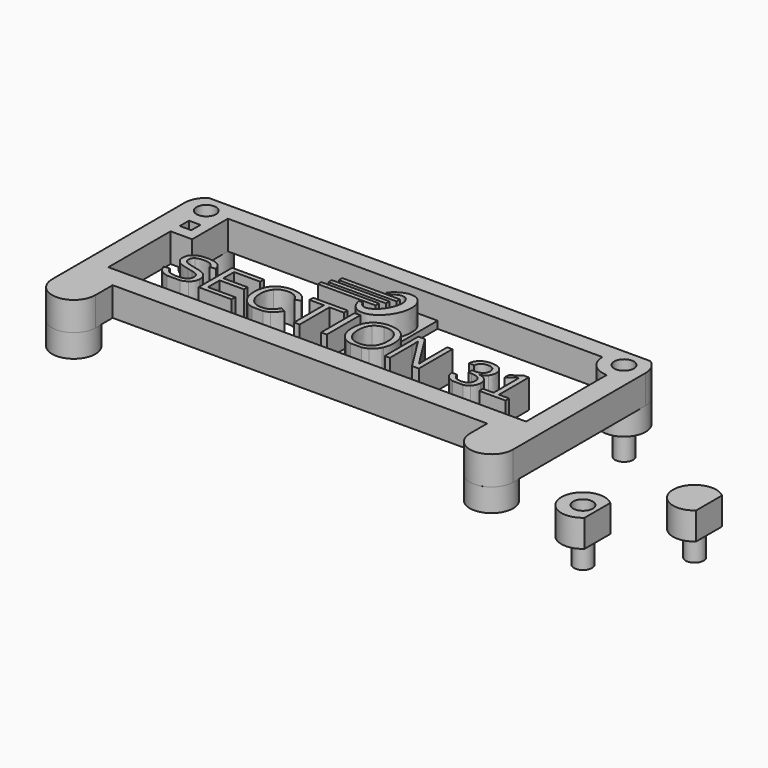
from build123d import *

# Parameters (mm, degrees)
F0_R      = 1.25
F1_DEPTH  = 3.8
F3_DEPTH  = 3.2
F0_R_2    = 3
F0_R_3    = 1.35
F4_W      = 0.7852271802
F4_H      = 1.481747925
F4_W_2    = 0.789192974
F4_W_3    = 0.7019455096
F4_H_2    = 4.3387154998
F4_W_4    = 0.7194174142
F4_H_3    = 0.6437805332
F4_W_5    = 2.3355792606
F4_H_4    = 0.6
F4_W_6    = 2.9250326228
F4_W_7    = 3.514485985
F5_DEPTH  = 1
F4_W_8    = 52
F4_H_5    = 3
F6_DEPTH  = 4
F4_W_9    = 5.6644207394
F4_W_10   = 5.0749673772
F4_W_11   = 4.485514015
F7_DEPTH  = 4
F8_R      = 1.35
F9_DEPTH  = 3
F10_DEPTH = 3.5
F2_R      = 1
F11_R     = 1.35
F11_R_2   = 1
F12_DEPTH = 2.5


with BuildPart() as f1:
    # F0 (on Top) → F1 (new body)
    with BuildSketch(Plane.XY):
        with BuildLine():
            Line((2, -2.2360679775), (2, 2.2360679775))
            ThreePointArc((2, 2.2360679775), (-3, 0), (2, -2.2360679775))
        make_face()
        Circle(F0_R, mode=Mode.SUBTRACT)
        Circle(F0_R)
    extrude(amount=F1_DEPTH)

    # F0 (on Top) → F10 (join)
    with BuildSketch(Plane.XY):
        Circle(F0_R)
    extrude(amount=-F10_DEPTH)

    # F2 (on face) + F11 (on face) → F12 (cut)
    with BuildSketch(Plane.XY.offset(3.8)):
        Circle(F2_R)
    with BuildSketch(Plane.XY.offset(3.8)):
        Circle(F11_R)
        Circle(F11_R_2, mode=Mode.SUBTRACT)
    extrude(amount=-F12_DEPTH, mode=Mode.SUBTRACT)


with BuildPart() as f1b:
    # F0 (on Top) → F1, piece 2 (new body)
    with BuildSketch(Plane.XY):
        with BuildLine():
            Line((10.3669340588, 6.6795249388), (10.3669340588, 11.1516608938))
            ThreePointArc((10.3669340588, 11.1516608938), (5.3669340588, 8.9155929163), (10.3669340588, 6.6795249388))
        make_face()
        with Locations((8.3669340588, 8.9155929163)):
            Circle(F0_R, mode=Mode.SUBTRACT)
        with Locations((8.3669340588, 8.9155929163)):
            Circle(F0_R)
    extrude(amount=F1_DEPTH)


with BuildPart() as f3:
    # F0 (on Top) → F3 (new body)
    with BuildSketch(Plane.XY):
        with BuildLine():
            Line((-11.3286585063, 25.8566533644), (-14.6452832967, 25.8566533644))
            ThreePointArc((-14.6452832967, 25.8566533644), (-12.9869709015, 20.3566533644), (-11.3286585063, 25.8566533644))
        make_face()
        with Locations((-12.9869709015, 23.3566533644)):
            Circle(F0_R, mode=Mode.SUBTRACT)
        with Locations((-12.9869709015, 23.3566533644)):
            Circle(F0_R)
    extrude(amount=F3_DEPTH)


with BuildPart() as f3b:
    # F0 (on Top) → F3, piece 2 (new body)
    with BuildSketch(Plane.XY):
        with BuildLine():
            Line((-69.3286585063, 25.8566533644), (-72.6452832967, 25.8566533644))
            ThreePointArc((-72.6452832967, 25.8566533644), (-70.9869709015, 20.3566533644), (-69.3286585063, 25.8566533644))
        make_face()
        with Locations((-70.9869709015, 23.3566533644)):
            Circle(F0_R, mode=Mode.SUBTRACT)
        with Locations((-70.9869709015, 23.3566533644)):
            Circle(F0_R)
    extrude(amount=F3_DEPTH)


with BuildPart() as f3c:
    # F0 (on Top) → F3, piece 3 (new body)
    with BuildSketch(Plane.XY):
        with Locations((-70.9869709015, 0.3566533644)):
            Circle(F0_R_2)
        with Locations((-70.9869709015, 0.3566533644)):
            Circle(F0_R_3, mode=Mode.SUBTRACT)
    extrude(amount=F3_DEPTH)


with BuildPart() as f3d:
    # F0 (on Top) → F3, piece 4 (new body)
    with BuildSketch(Plane.XY):
        with Locations((-12.9869709015, 0.3566533644)):
            Circle(F0_R_2)
        with Locations((-12.9869709015, 0.3566533644)):
            Circle(F0_R_3, mode=Mode.SUBTRACT)
    extrude(amount=F3_DEPTH)


with BuildPart() as f5:
    # F4 (on face) → F5 (new body)
    with BuildSketch(Plane.XY.offset(3.2)):
        with BuildLine():
            Line((-65.9445128975, 10.2926716208), (-70.9869709015, 10.2926716208))
            Line((-70.9869709015, 10.2926716208), (-70.9869709015, 8.8109236958))
            Line((-70.9869709015, 8.8109236958), (-64.8152467128, 8.8109236958))
            add(Edge.make_bspline(
                [(-64.8152467128, 8.8109236958), (-66.1138597254, 9.0786315838), (-66.3719762536, 10.2068831272)],
                knots=[0.2372767753, 0.2372767753, 0.2372767753, 1, 1, 1], degree=2))
            Line((-66.3719762536, 10.2068831272), (-65.9445128975, 10.2926716208))
        make_face()
        with BuildLine():
            Line((-65.58930585, 10.2926716208), (-65.9445128975, 10.2926716208))
            Line((-65.9445128975, 10.2926716208), (-66.3719762536, 10.2068831272))
            add(Edge.make_bspline(
                [(-64.8152467128, 8.8109236958), (-66.1138597254, 9.0786315838), (-66.3719762536, 10.2068831272)],
                knots=[0.2372767753, 0.2372767753, 0.2372767753, 1, 1, 1], degree=2))
            Line((-64.8152467128, 8.8109236958), (-63.0099098319, 8.8109236958))
            add(Edge.make_bspline(
                [(-62.1318816738, 9.1698280383), (-62.4884162435, 8.919543015), (-63.0099098319, 8.8109236958)],
                knots=[0, 0, 0, 0.5660175036, 0.5660175036, 0.5660175036], degree=2))
            add(Edge.make_bspline(
                [(-61.5059502002, 10.2926716208), (-61.5519807819, 9.5769148133), (-62.1318816738, 9.1698280383)],
                knots=[0.0793766355, 0.0793766355, 0.0793766355, 1, 1, 1], degree=2))
            Line((-61.5059502002, 10.2926716208), (-62.2861622514, 10.2926716208))
            add(Edge.make_bspline(
                [(-62.6983292272, 9.6060653606), (-62.3180540452, 9.8464622511), (-62.2861622514, 10.2926716208)],
                knots=[0, 0, 0, 0.9161349587, 0.9161349587, 0.9161349587], degree=2))
            add(Edge.make_bspline(
                [(-63.8774919287, 9.3436620015), (-63.113415649, 9.3436620015), (-62.6983292272, 9.6060653606)],
                knots=[0, 0, 0, 1, 1, 1], degree=2))
            add(Edge.make_bspline(
                [(-65.04607918, 9.5895412196), (-64.6164515141, 9.3436620015), (-63.8774919287, 9.3436620015)],
                knots=[0, 0, 0, 1, 1, 1], degree=2))
            add(Edge.make_bspline(
                [(-65.58930585, 10.2926716208), (-65.4475651637, 9.8193147364), (-65.04607918, 9.5895412196)],
                knots=[0.0655024909, 0.0655024909, 0.0655024909, 1, 1, 1], degree=2))
        make_face()
        with BuildLine():
            Line((-62.2861622514, 10.2926716208), (-65.58930585, 10.2926716208))
            add(Edge.make_bspline(
                [(-65.58930585, 10.2926716208), (-65.4475651637, 9.8193147364), (-65.04607918, 9.5895412196)],
                knots=[0.0655024909, 0.0655024909, 0.0655024909, 1, 1, 1], degree=2))
            add(Edge.make_bspline(
                [(-65.04607918, 9.5895412196), (-64.6164515141, 9.3436620015), (-63.8774919287, 9.3436620015)],
                knots=[0, 0, 0, 1, 1, 1], degree=2))
            add(Edge.make_bspline(
                [(-63.8774919287, 9.3436620015), (-63.113415649, 9.3436620015), (-62.6983292272, 9.6060653606)],
                knots=[0, 0, 0, 1, 1, 1], degree=2))
            add(Edge.make_bspline(
                [(-62.6983292272, 9.6060653606), (-62.3180540452, 9.8464622511), (-62.2861622514, 10.2926716208)],
                knots=[0, 0, 0, 0.9161349587, 0.9161349587, 0.9161349587], degree=2))
        make_face()
        with BuildLine():
            add(Edge.make_bspline(
                [(-62.1318816738, 9.1698280383), (-62.4884162435, 8.919543015), (-63.0099098319, 8.8109236958)],
                knots=[0, 0, 0, 0.5660175036, 0.5660175036, 0.5660175036], degree=2))
            Line((-63.0099098319, 8.8109236958), (-60.4193197009, 8.8109236958))
            Line((-60.4193197009, 8.8109236958), (-60.4193197009, 10.2926716208))
            Line((-60.4193197009, 10.2926716208), (-61.5059502002, 10.2926716208))
            add(Edge.make_bspline(
                [(-61.5059502002, 10.2926716208), (-61.5519807819, 9.5769148133), (-62.1318816738, 9.1698280383)],
                knots=[0.0793766355, 0.0793766355, 0.0793766355, 1, 1, 1], degree=2))
        make_face()
        Polygon((-60.4193197009, 10.2926716208), (-60.4193197009, 8.8109236958), (-55.8335400914, 8.8109236958), (-55.8335400914, 9.4560261603), (-59.6301267269, 9.4560261603), (-59.6301267269, 10.2926716208), align=None)
        with BuildLine():
            Line((-55.8335400914, 9.4560261603), (-55.8335400914, 8.8109236958))
            Line((-55.8335400914, 8.8109236958), (-52.9878142088, 8.8109236958))
            add(Edge.make_bspline(
                [(-52.9878142088, 8.8109236958), (-53.3889917697, 8.9022720993), (-53.7250597001, 9.0938169897)],
                knots=[0.4769033687, 0.4769033687, 0.4769033687, 1, 1, 1], degree=2))
            add(Edge.make_bspline(
                [(-53.7250597001, 9.0938169897), (-54.3675183021, 9.4599919542), (-54.7039498128, 10.139464632)],
                knots=[0, 0, 0, 1, 1, 1], degree=2))
            add(Edge.make_bspline(
                [(-54.7039498128, 10.139464632), (-54.7411237954, 10.2145429308), (-54.7741902407, 10.2926716208)],
                knots=[0, 0, 0, 0.110494949, 0.110494949, 0.110494949], degree=2))
            Line((-54.7741902407, 10.2926716208), (-59.6301267269, 10.2926716208))
            Line((-59.6301267269, 10.2926716208), (-59.6301267269, 9.4560261603))
            Line((-59.6301267269, 9.4560261603), (-55.8335400914, 9.4560261603))
        make_face()
        with BuildLine():
            add(Edge.make_bspline(
                [(-52.9878142088, 8.8109236958), (-53.3889917697, 8.9022720993), (-53.7250597001, 9.0938169897)],
                knots=[0.4769033687, 0.4769033687, 0.4769033687, 1, 1, 1], degree=2))
            Line((-52.9878142088, 8.8109236958), (-51.4550116902, 8.8109236958))
            add(Edge.make_bspline(
                [(-50.6925493444, 9.1202556153), (-51.0433918047, 8.9084665691), (-51.4550116902, 8.8109236958)],
                knots=[0, 0, 0, 0.5394338135, 0.5394338135, 0.5394338135], degree=2))
            add(Edge.make_bspline(
                [(-49.6825938466, 10.2650481035), (-50.0421591547, 9.5128692054), (-50.6925493444, 9.1202556153)],
                knots=[0, 0, 0, 1, 1, 1], degree=2))
            Line((-49.6825938466, 10.2650481035), (-49.7377276701, 10.2926716208))
            Line((-49.7377276701, 10.2926716208), (-50.4971638043, 10.2926716208))
            add(Edge.make_bspline(
                [(-52.16518079, 9.3767102835), (-51.101681984, 9.3767102835), (-50.4971638043, 10.2926716208)],
                knots=[0, 0, 0, 0.8697338936, 0.8697338936, 0.8697338936], degree=2))
            add(Edge.make_bspline(
                [(-53.679453071, 10.0277614388), (-53.119615174, 9.3767102835), (-52.16518079, 9.3767102835)],
                knots=[0, 0, 0, 1, 1, 1], degree=2))
            add(Edge.make_bspline(
                [(-53.8734730775, 10.2926716208), (-53.7867440439, 10.1525331133), (-53.679453071, 10.0277614388)],
                knots=[0.8083535011, 0.8083535011, 0.8083535011, 1, 1, 1], degree=2))
            Line((-53.8734730775, 10.2926716208), (-54.7741902407, 10.2926716208))
            add(Edge.make_bspline(
                [(-54.7039498128, 10.139464632), (-54.7411237954, 10.2145429308), (-54.7741902407, 10.2926716208)],
                knots=[0, 0, 0, 0.110494949, 0.110494949, 0.110494949], degree=2))
            add(Edge.make_bspline(
                [(-53.7250597001, 9.0938169897), (-54.3675183021, 9.4599919542), (-54.7039498128, 10.139464632)],
                knots=[0, 0, 0, 1, 1, 1], degree=2))
        make_face()
        with BuildLine():
            add(Edge.make_bspline(
                [(-52.16518079, 9.3767102835), (-51.101681984, 9.3767102835), (-50.4971638043, 10.2926716208)],
                knots=[0, 0, 0, 0.8697338936, 0.8697338936, 0.8697338936], degree=2))
            Line((-50.4971638043, 10.2926716208), (-53.8734730775, 10.2926716208))
            add(Edge.make_bspline(
                [(-53.8734730775, 10.2926716208), (-53.7867440439, 10.1525331133), (-53.679453071, 10.0277614388)],
                knots=[0.8083535011, 0.8083535011, 0.8083535011, 1, 1, 1], degree=2))
            add(Edge.make_bspline(
                [(-53.679453071, 10.0277614388), (-53.119615174, 9.3767102835), (-52.16518079, 9.3767102835)],
                knots=[0, 0, 0, 1, 1, 1], degree=2))
        make_face()
        with BuildLine():
            Line((-47.1709244151, 8.8109236958), (-47.1709244151, 10.2926716208))
            Line((-47.1709244151, 10.2926716208), (-49.7377276701, 10.2926716208))
            Line((-49.7377276701, 10.2926716208), (-49.6825938466, 10.2650481035))
            add(Edge.make_bspline(
                [(-49.6825938466, 10.2650481035), (-50.0421591547, 9.5128692054), (-50.6925493444, 9.1202556153)],
                knots=[0, 0, 0, 1, 1, 1], degree=2))
            add(Edge.make_bspline(
                [(-50.6925493444, 9.1202556153), (-51.0433918047, 8.9084665691), (-51.4550116902, 8.8109236958)],
                knots=[0, 0, 0, 0.5394338135, 0.5394338135, 0.5394338135], degree=2))
            Line((-51.4550116902, 8.8109236958), (-47.1709244151, 8.8109236958))
        make_face()
        with Locations((-46.778310825, 9.5517976583)):
            Rectangle(F4_W, F4_H)
        Polygon((-43.4113518554, 8.8109236958), (-43.4113518554, 10.2926716208), (-45.1050326228, 10.2926716208), (-46.3856972349, 10.2926716208), (-46.3856972349, 8.8109236958), align=None)
        with Locations((-43.0167553684, 9.5517976583)):
            Rectangle(F4_W_2, F4_H)
        with BuildLine():
            add(Edge.make_bspline(
                [(-41.0986330815, 10.1434304258), (-41.1352188102, 10.2167428687), (-41.1679026296, 10.2926716208)],
                knots=[0, 0, 0, 0.1066511318, 0.1066511318, 0.1066511318], degree=2))
            Line((-41.1679026296, 10.2926716208), (-42.6221588814, 10.2926716208))
            Line((-42.6221588814, 10.2926716208), (-42.6221588814, 8.8109236958))
            Line((-42.6221588814, 8.8109236958), (-39.3595075306, 8.8109236958))
            add(Edge.make_bspline(
                [(-39.3595075306, 8.8109236958), (-39.7658280531, 8.9017986323), (-40.1052017247, 9.0918340928)],
                knots=[0.4781998914, 0.4781998914, 0.4781998914, 1, 1, 1], degree=2))
            add(Edge.make_bspline(
                [(-40.1052017247, 9.0918340928), (-40.7555919144, 9.4560261603), (-41.0986330815, 10.1434304258)],
                knots=[0, 0, 0, 1, 1, 1], degree=2))
        make_face()
        with BuildLine():
            add(Edge.make_bspline(
                [(-40.2911840801, 10.2926716208), (-40.2014529772, 10.1425159595), (-40.0886775837, 10.0112372978)],
                knots=[0.7956620687, 0.7956620687, 0.7956620687, 1, 1, 1], degree=2))
            Line((-40.2911840801, 10.2926716208), (-41.1679026296, 10.2926716208))
            add(Edge.make_bspline(
                [(-41.0986330815, 10.1434304258), (-41.1352188102, 10.2167428687), (-41.1679026296, 10.2926716208)],
                knots=[0, 0, 0, 0.1066511318, 0.1066511318, 0.1066511318], degree=2))
            add(Edge.make_bspline(
                [(-40.1052017247, 9.0918340928), (-40.7555919144, 9.4560261603), (-41.0986330815, 10.1434304258)],
                knots=[0, 0, 0, 1, 1, 1], degree=2))
            add(Edge.make_bspline(
                [(-39.3595075306, 8.8109236958), (-39.7658280531, 8.9017986323), (-40.1052017247, 9.0918340928)],
                knots=[0.4781998914, 0.4781998914, 0.4781998914, 1, 1, 1], degree=2))
            Line((-39.3595075306, 8.8109236958), (-37.7667528951, 8.8109236958))
            add(Edge.make_bspline(
                [(-37.0171702552, 9.0957998866), (-37.359609992, 8.902744286), (-37.7667528951, 8.8109236958)],
                knots=[0, 0, 0, 0.5243826652, 0.5243826652, 0.5243826652], degree=2))
            add(Edge.make_bspline(
                [(-36.0151463452, 10.1493791166), (-36.364136203, 9.463957748), (-37.0171702552, 9.0957998866)],
                knots=[0, 0, 0, 1, 1, 1], degree=2))
            add(Edge.make_bspline(
                [(-35.9470997448, 10.2926716208), (-35.9792800212, 10.2198211202), (-36.0151463452, 10.1493791166)],
                knots=[0.8972281769, 0.8972281769, 0.8972281769, 1, 1, 1], degree=2))
            Line((-35.9470997448, 10.2926716208), (-36.7974095037, 10.2926716208))
            add(Edge.make_bspline(
                [(-37.0105605988, 9.990747363), (-36.8906570495, 10.1290184903), (-36.7974095037, 10.2926716208)],
                knots=[0, 0, 0, 0.2223120466, 0.2223120466, 0.2223120466], degree=2))
            add(Edge.make_bspline(
                [(-38.5585421274, 9.3687786959), (-37.549908561, 9.3687786959), (-37.0105605988, 9.990747363)],
                knots=[0, 0, 0, 1, 1, 1], degree=2))
            add(Edge.make_bspline(
                [(-40.0886775837, 10.0112372978), (-39.5367712744, 9.3687786959), (-38.5585421274, 9.3687786959)],
                knots=[0, 0, 0, 1, 1, 1], degree=2))
        make_face()
        with BuildLine():
            Line((-36.7974095037, 10.2926716208), (-38.8689091802, 10.2926716208))
            Line((-38.8689091802, 10.2926716208), (-40.2911840801, 10.2926716208))
            add(Edge.make_bspline(
                [(-40.2911840801, 10.2926716208), (-40.2014529772, 10.1425159595), (-40.0886775837, 10.0112372978)],
                knots=[0.7956620687, 0.7956620687, 0.7956620687, 1, 1, 1], degree=2))
            add(Edge.make_bspline(
                [(-40.0886775837, 10.0112372978), (-39.5367712744, 9.3687786959), (-38.5585421274, 9.3687786959)],
                knots=[0, 0, 0, 1, 1, 1], degree=2))
            add(Edge.make_bspline(
                [(-38.5585421274, 9.3687786959), (-37.549908561, 9.3687786959), (-37.0105605988, 9.990747363)],
                knots=[0, 0, 0, 1, 1, 1], degree=2))
            add(Edge.make_bspline(
                [(-37.0105605988, 9.990747363), (-36.8906570495, 10.1290184903), (-36.7974095037, 10.2926716208)],
                knots=[0, 0, 0, 0.2223120466, 0.2223120466, 0.2223120466], degree=2))
        make_face()
        with BuildLine():
            Line((-34.5676315938, 10.2926716208), (-35.9470997448, 10.2926716208))
            add(Edge.make_bspline(
                [(-35.9470997448, 10.2926716208), (-35.9792800212, 10.2198211202), (-36.0151463452, 10.1493791166)],
                knots=[0.8972281769, 0.8972281769, 0.8972281769, 1, 1, 1], degree=2))
            add(Edge.make_bspline(
                [(-36.0151463452, 10.1493791166), (-36.364136203, 9.463957748), (-37.0171702552, 9.0957998866)],
                knots=[0, 0, 0, 1, 1, 1], degree=2))
            add(Edge.make_bspline(
                [(-37.0171702552, 9.0957998866), (-37.359609992, 8.902744286), (-37.7667528951, 8.8109236958)],
                knots=[0, 0, 0, 0.5243826652, 0.5243826652, 0.5243826652], degree=2))
            Line((-37.7667528951, 8.8109236958), (-34.5676315938, 8.8109236958))
            Line((-34.5676315938, 8.8109236958), (-34.5676315938, 10.2926716208))
        make_face()
        with Locations((-34.216658839, 9.5517976583)):
            Rectangle(F4_W_3, F4_H)
        Polygon((-31.7231286885, 10.2926716208), (-33.8656860843, 10.2926716208), (-33.8656860843, 8.8109236958), (-30.7921958588, 8.8109236958), align=None)
        with BuildLine():
            Line((-30.7921958588, 8.8109236958), (-29.8417272687, 8.8109236958))
            Line((-29.8417272687, 8.8109236958), (-29.8417272687, 10.2926716208))
            Line((-29.8417272687, 10.2926716208), (-30.5373681675, 10.2926716208))
            add(Edge.make_bspline(
                [(-30.5026929085, 9.6410965395), (-30.5252166185, 10.0142596264), (-30.5373681675, 10.2926716208)],
                knots=[0, 0, 0, 0.4604996702, 0.4604996702, 0.4604996702], degree=2))
            Line((-30.5026929085, 9.6410965395), (-30.9136598671, 10.2926716208))
            Line((-30.9136598671, 10.2926716208), (-31.7231286885, 10.2926716208))
            Line((-31.7231286885, 10.2926716208), (-30.7921958588, 8.8109236958))
        make_face()
        with BuildLine():
            add(Edge.make_bspline(
                [(-30.5026929085, 9.6410965395), (-30.5252166185, 10.0142596264), (-30.5373681675, 10.2926716208)],
                knots=[0, 0, 0, 0.4604996702, 0.4604996702, 0.4604996702], degree=2))
            Line((-30.5373681675, 10.2926716208), (-30.9136598671, 10.2926716208))
            Line((-30.9136598671, 10.2926716208), (-30.5026929085, 9.6410965395))
        make_face()
        with BuildLine():
            Line((-29.8417272687, 8.8109236958), (-25.1752851151, 8.8109236958))
            add(Edge.make_bspline(
                [(-25.1752851151, 8.8109236958), (-25.5666146624, 8.9099823085), (-25.852799632, 9.1268652717)],
                knots=[0.4567376397, 0.4567376397, 0.4567376397, 1, 1, 1], degree=2))
            add(Edge.make_bspline(
                [(-25.852799632, 9.1268652717), (-26.3750691824, 9.5226630238), (-26.4770012039, 10.2926716208)],
                knots=[0, 0, 0, 0.991419602, 0.991419602, 0.991419602], degree=2))
            Line((-26.4770012039, 10.2926716208), (-29.8417272687, 10.2926716208))
            Line((-29.8417272687, 10.2926716208), (-29.8417272687, 8.8109236958))
        make_face()
        with BuildLine():
            add(Edge.make_bspline(
                [(-23.5605707929, 9.6206066047), (-23.285597977, 9.8581604394), (-23.2464876626, 10.2926716208)],
                knots=[0, 0, 0, 0.8577666151, 0.8577666151, 0.8577666151], degree=2))
            Line((-23.2464876626, 10.2926716208), (-25.6967195206, 10.2926716208))
            add(Edge.make_bspline(
                [(-25.6967195206, 10.2926716208), (-25.5151816234, 9.3436620015), (-24.4429599221, 9.3436620015)],
                knots=[0.0412500578, 0.0412500578, 0.0412500578, 1, 1, 1], degree=2))
            add(Edge.make_bspline(
                [(-24.4429599221, 9.3436620015), (-23.8811391282, 9.3436620015), (-23.5605707929, 9.6206066047)],
                knots=[0, 0, 0, 1, 1, 1], degree=2))
        make_face()
        with BuildLine():
            add(Edge.make_bspline(
                [(-22.471222088, 10.2926716208), (-22.5086551424, 9.5769148133), (-22.9802429611, 9.1698280383)],
                knots=[0.0793766355, 0.0793766355, 0.0793766355, 1, 1, 1], degree=2))
            Line((-22.471222088, 10.2926716208), (-23.2464876626, 10.2926716208))
            add(Edge.make_bspline(
                [(-23.5605707929, 9.6206066047), (-23.285597977, 9.8581604394), (-23.2464876626, 10.2926716208)],
                knots=[0, 0, 0, 0.8577666151, 0.8577666151, 0.8577666151], degree=2))
            add(Edge.make_bspline(
                [(-24.4429599221, 9.3436620015), (-23.8811391282, 9.3436620015), (-23.5605707929, 9.6206066047)],
                knots=[0, 0, 0, 1, 1, 1], degree=2))
            add(Edge.make_bspline(
                [(-25.6967195206, 10.2926716208), (-25.5151816234, 9.3436620015), (-24.4429599221, 9.3436620015)],
                knots=[0.0412500578, 0.0412500578, 0.0412500578, 1, 1, 1], degree=2))
            Line((-25.6967195206, 10.2926716208), (-26.4770012039, 10.2926716208))
            add(Edge.make_bspline(
                [(-25.852799632, 9.1268652717), (-26.3750691824, 9.5226630238), (-26.4770012039, 10.2926716208)],
                knots=[0, 0, 0, 0.991419602, 0.991419602, 0.991419602], degree=2))
            add(Edge.make_bspline(
                [(-25.1752851151, 8.8109236958), (-25.5666146624, 8.9099823085), (-25.852799632, 9.1268652717)],
                knots=[0.4567376397, 0.4567376397, 0.4567376397, 1, 1, 1], degree=2))
            Line((-25.1752851151, 8.8109236958), (-23.7005212089, 8.8109236958))
            add(Edge.make_bspline(
                [(-22.9802429611, 9.1698280383), (-23.2701845052, 8.919543015), (-23.7005212089, 8.8109236958)],
                knots=[0, 0, 0, 0.5660175036, 0.5660175036, 0.5660175036], degree=2))
        make_face()
        with BuildLine():
            Line((-19.9695444714, 9.4428068475), (-19.9695444714, 10.2926716208))
            Line((-19.9695444714, 10.2926716208), (-22.471222088, 10.2926716208))
            add(Edge.make_bspline(
                [(-22.471222088, 10.2926716208), (-22.5086551424, 9.5769148133), (-22.9802429611, 9.1698280383)],
                knots=[0.0793766355, 0.0793766355, 0.0793766355, 1, 1, 1], degree=2))
            add(Edge.make_bspline(
                [(-22.9802429611, 9.1698280383), (-23.2701845052, 8.919543015), (-23.7005212089, 8.8109236958)],
                knots=[0, 0, 0, 0.5660175036, 0.5660175036, 0.5660175036], degree=2))
            Line((-23.7005212089, 8.8109236958), (-21.451429436, 8.8109236958))
            Line((-21.451429436, 8.8109236958), (-21.451429436, 9.4428068475))
            Line((-21.451429436, 9.4428068475), (-19.9695444714, 9.4428068475))
        make_face()
        Polygon((-19.221331367, 9.4428068475), (-19.221331367, 10.2926716208), (-19.9695444714, 10.2926716208), (-19.9695444714, 9.4428068475), (-21.451429436, 9.4428068475), (-21.451429436, 8.8109236958), (-17.8042210351, 8.8109236958), (-17.8042210351, 9.4428068475), align=None)
        Polygon((-12.9869709015, 8.8109236958), (-12.9869709015, 10.2926716208), (-19.221331367, 10.2926716208), (-19.221331367, 9.4428068475), (-17.8042210351, 9.4428068475), (-17.8042210351, 8.8109236958), align=None)
        with BuildLine():
            Line((-38.8689091802, 14.7072367602), (-38.8689091802, 23.3566533644))
            Line((-38.8689091802, 23.3566533644), (-45.1050326228, 23.3566533644))
            Line((-45.1050326228, 23.3566533644), (-45.1050326228, 20.2072403342))
            Line((-45.1050326228, 20.2072403342), (-41.5905466378, 20.2072403342))
            Line((-41.5905466378, 20.2072403342), (-41.5905466378, 19.6072403342))
            Line((-41.5905466378, 19.6072403342), (-45.1050326228, 19.6072403342))
            Line((-45.1050326228, 19.6072403342), (-45.1050326228, 19.13))
            Line((-45.1050326228, 19.13), (-42.18, 19.13))
            Line((-42.18, 19.13), (-42.18, 18.53))
            Line((-42.18, 18.53), (-45.1050326228, 18.53))
            Line((-45.1050326228, 18.53), (-45.1050326228, 18.0527596658))
            Line((-45.1050326228, 18.0527596658), (-42.7694533622, 18.0527596658))
            Line((-42.7694533622, 18.0527596658), (-42.7694533622, 17.4527596658))
            Line((-42.7694533622, 17.4527596658), (-45.1050326228, 17.4527596658))
            Line((-45.1050326228, 17.4527596658), (-45.1050326228, 14.6313871206))
            Line((-45.1050326228, 14.6313871206), (-44.3856152086, 14.6313871206))
            Line((-44.3856152086, 14.6313871206), (-44.3856152086, 13.9876065874))
            Line((-44.3856152086, 13.9876065874), (-45.1050326228, 13.9876065874))
            Line((-45.1050326228, 13.9876065874), (-45.1050326228, 10.2926716208))
            Line((-45.1050326228, 10.2926716208), (-43.4113518554, 10.2926716208))
            Line((-43.4113518554, 10.2926716208), (-43.4113518554, 14.6313871206))
            Line((-43.4113518554, 14.6313871206), (-42.6221588814, 14.6313871206))
            Line((-42.6221588814, 14.6313871206), (-42.6221588814, 10.2926716208))
            Line((-42.6221588814, 10.2926716208), (-41.1679026296, 10.2926716208))
            add(Edge.make_bspline(
                [(-41.1679026296, 10.2926716208), (-41.4416742486, 10.9286786055), (-41.4416742486, 11.7482549994)],
                knots=[0.1066511318, 0.1066511318, 0.1066511318, 1, 1, 1], degree=2))
            add(Edge.make_bspline(
                [(-41.4416742486, 11.7482549994), (-41.4416742486, 13.1442144309), (-40.6775979689, 13.931424508)],
                knots=[0, 0, 0, 1, 1, 1], degree=2))
            add(Edge.make_bspline(
                [(-40.6775979689, 13.931424508), (-40.0054612416, 14.6239113956), (-38.8689091802, 14.7072367602)],
                knots=[0, 0, 0, 0.8796722855, 0.8796722855, 0.8796722855], degree=2))
        make_face()
        with BuildLine():
            add(Edge.make_bspline(
                [(-44.806121809, 17.1282714965), (-43.205691342, 6.4668306235), (-39.5316900865, 18.1957354999), (-35.857688831, 29.9246403764), (-43.7372763612, 20.5404604734)],
                knots=[2.3784830967, 2.3784830967, 2.3784830967, 4.9739426441, 4.9739426441, 7.5694021915, 7.5694021915, 7.5694021915], degree=2, weights=[1, 0.2696856325, 1, 0.2696856325, 1]))
            Line((-44.806121809, 17.1282714965), (-44.2693105322, 17.1282714965))
            add(Edge.make_bspline(
                [(-44.2693105322, 17.1282714965), (-42.999690023, 13.2713551301), (-41.040963668, 18.4754613686), (-39.0822373129, 23.679567607), (-42.9850276657, 20.5404604734)],
                knots=[2.6230590625, 2.6230590625, 2.6230590625, 4.9309827595, 4.9309827595, 7.2389064564, 7.2389064564, 7.2389064564], degree=2, weights=[1, 0.4048680121, 1, 0.4048680121, 1]))
            Line((-42.9850276657, 20.5404604734), (-43.7372763612, 20.5404604734))
        make_face(mode=Mode.SUBTRACT)
        with BuildLine():
            Line((-38.8689091802, 10.2926716208), (-38.8689091802, 14.0566915167))
            add(Edge.make_bspline(
                [(-38.8689091802, 14.0566915167), (-39.6404911653, 13.9720617755), (-40.0952872401, 13.4621389036)],
                knots=[0.1659657684, 0.1659657684, 0.1659657684, 1, 1, 1], degree=2))
            add(Edge.make_bspline(
                [(-40.0952872401, 13.4621389036), (-40.6405838931, 12.8507456868), (-40.6405838931, 11.7482549994)],
                knots=[0, 0, 0, 1, 1, 1], degree=2))
            add(Edge.make_bspline(
                [(-40.6405838931, 11.7482549994), (-40.6405838931, 10.8773558419), (-40.2911840801, 10.2926716208)],
                knots=[0, 0, 0, 0.7956620687, 0.7956620687, 0.7956620687], degree=2))
            Line((-40.2911840801, 10.2926716208), (-38.8689091802, 10.2926716208))
        make_face()
        with BuildLine():
            Line((-38.8689091802, 14.0566915167), (-38.8689091802, 14.7072367602))
            add(Edge.make_bspline(
                [(-40.6775979689, 13.931424508), (-40.0054612416, 14.6239113956), (-38.8689091802, 14.7072367602)],
                knots=[0, 0, 0, 0.8796722855, 0.8796722855, 0.8796722855], degree=2))
            add(Edge.make_bspline(
                [(-41.4416742486, 11.7482549994), (-41.4416742486, 13.1442144309), (-40.6775979689, 13.931424508)],
                knots=[0, 0, 0, 1, 1, 1], degree=2))
            add(Edge.make_bspline(
                [(-41.1679026296, 10.2926716208), (-41.4416742486, 10.9286786055), (-41.4416742486, 11.7482549994)],
                knots=[0.1066511318, 0.1066511318, 0.1066511318, 1, 1, 1], degree=2))
            Line((-41.1679026296, 10.2926716208), (-40.2911840801, 10.2926716208))
            add(Edge.make_bspline(
                [(-40.6405838931, 11.7482549994), (-40.6405838931, 10.8773558419), (-40.2911840801, 10.2926716208)],
                knots=[0, 0, 0, 0.7956620687, 0.7956620687, 0.7956620687], degree=2))
            add(Edge.make_bspline(
                [(-40.0952872401, 13.4621389036), (-40.6405838931, 12.8507456868), (-40.6405838931, 11.7482549994)],
                knots=[0, 0, 0, 1, 1, 1], degree=2))
            add(Edge.make_bspline(
                [(-38.8689091802, 14.0566915167), (-39.6404911653, 13.9720617755), (-40.0952872401, 13.4621389036)],
                knots=[0.1659657684, 0.1659657684, 0.1659657684, 1, 1, 1], degree=2))
        make_face()
        with Locations((-43.0167553684, 12.4620293707)):
            Rectangle(F4_W_2, F4_H_2)
        with Locations((-44.7453239157, 14.309496854)):
            Rectangle(F4_W_4, F4_H_3)
        with BuildLine():
            Line((-44.2693105322, 17.1282714965), (-44.806121809, 17.1282714965))
            add(Edge.make_bspline(
                [(-44.806121809, 17.1282714965), (-43.205691342, 6.4668306235), (-39.5316900865, 18.1957354999), (-35.857688831, 29.9246403764), (-43.7372763612, 20.5404604734)],
                knots=[2.3784830967, 2.3784830967, 2.3784830967, 4.9739426441, 4.9739426441, 7.5694021915, 7.5694021915, 7.5694021915], degree=2, weights=[1, 0.2696856325, 1, 0.2696856325, 1]))
            Line((-43.7372763612, 20.5404604734), (-42.9850276657, 20.5404604734))
            add(Edge.make_bspline(
                [(-44.2693105322, 17.1282714965), (-42.999690023, 13.2713551301), (-41.040963668, 18.4754613686), (-39.0822373129, 23.679567607), (-42.9850276657, 20.5404604734)],
                knots=[2.6230590625, 2.6230590625, 2.6230590625, 4.9309827595, 4.9309827595, 7.2389064564, 7.2389064564, 7.2389064564], degree=2, weights=[1, 0.4048680121, 1, 0.4048680121, 1]))
        make_face()
        with Locations((-43.9372429925, 17.7527596658)):
            Rectangle(F4_W_5, F4_H_4)
        with Locations((-43.6425163114, 18.83)):
            Rectangle(F4_W_6, F4_H_4)
        with Locations((-43.3477896303, 19.9072403342)):
            Rectangle(F4_W_7, F4_H_4)
    extrude(amount=F5_DEPTH)


with BuildPart() as f6:
    # F4 (on face) → F6 (new body)
    with BuildSketch(Plane.XY.offset(3.2)):
        with BuildLine():
            ThreePointArc((-9.9869709015, 23.3566533644), (-10.8656505579, 21.2353330208), (-12.9869709015, 20.3566533644))
            Line((-12.9869709015, 20.3566533644), (-12.9869709015, 10.2926716208))
            Line((-12.9869709015, 10.2926716208), (-12.9869709015, 8.8109236958))
            Line((-12.9869709015, 8.8109236958), (-12.9869709015, 6.3566533644))
            Line((-12.9869709015, 6.3566533644), (-15.9869709015, 6.3566533644))
            Line((-15.9869709015, 6.3566533644), (-15.9869709015, 3.3566533644))
            Line((-15.9869709015, 3.3566533644), (-15.9869709015, 0.3566533644))
            ThreePointArc((-15.9869709015, 0.3566533644), (-12.9869709015, 3.3566533644), (-9.9869709015, 0.3566533644))
            Line((-9.9869709015, 0.3566533644), (-9.9869709015, 23.3566533644))
        make_face()
        with BuildLine():
            ThreePointArc((-15.9869709015, 0.3566533644), (-12.9869709015, -2.6433466356), (-9.9869709015, 0.3566533644))
            ThreePointArc((-9.9869709015, 0.3566533644), (-12.9869709015, 3.3566533644), (-15.9869709015, 0.3566533644))
        make_face()
        with BuildLine():
            Line((-11.3286585063, 25.8566533644), (-14.6452832967, 25.8566533644))
            ThreePointArc((-14.6452832967, 25.8566533644), (-15.6303529383, 24.7752905298), (-15.9869709015, 23.3566533644))
            ThreePointArc((-15.9869709015, 23.3566533644), (-15.108291245, 21.2353330208), (-12.9869709015, 20.3566533644))
            ThreePointArc((-12.9869709015, 20.3566533644), (-10.8656505579, 21.2353330208), (-9.9869709015, 23.3566533644))
            ThreePointArc((-9.9869709015, 23.3566533644), (-10.3435888646, 24.7752905298), (-11.3286585063, 25.8566533644))
        make_face()
        with BuildLine():
            ThreePointArc((-15.9869709015, 23.3566533644), (-15.6303529383, 24.7752905298), (-14.6452832967, 25.8566533644))
            Line((-14.6452832967, 25.8566533644), (-69.3286585063, 25.8566533644))
            ThreePointArc((-69.3286585063, 25.8566533644), (-68.3435888646, 24.7752905298), (-67.9869709015, 23.3566533644))
            Line((-67.9869709015, 23.3566533644), (-45.1050326228, 23.3566533644))
            Line((-45.1050326228, 23.3566533644), (-38.8689091802, 23.3566533644))
            Line((-38.8689091802, 23.3566533644), (-15.9869709015, 23.3566533644))
        make_face()
        with BuildLine():
            ThreePointArc((-67.9869709015, 23.3566533644), (-68.3435888646, 24.7752905298), (-69.3286585063, 25.8566533644))
            Line((-69.3286585063, 25.8566533644), (-72.6452832967, 25.8566533644))
            ThreePointArc((-72.6452832967, 25.8566533644), (-73.6303529383, 24.7752905298), (-73.9869709015, 23.3566533644))
            ThreePointArc((-73.9869709015, 23.3566533644), (-73.108291245, 21.2353330208), (-70.9869709015, 20.3566533644))
            ThreePointArc((-70.9869709015, 20.3566533644), (-70.154248416, 20.4745407257), (-69.3869709015, 20.8189378563))
            ThreePointArc((-69.3869709015, 20.8189378563), (-68.3601857942, 21.9075156898), (-67.9869709015, 23.3566533644))
        make_face()
        with BuildLine():
            ThreePointArc((-70.9869709015, 20.3566533644), (-73.108291245, 21.2353330208), (-73.9869709015, 23.3566533644))
            Line((-73.9869709015, 23.3566533644), (-73.9869709015, 0.3566533644))
            ThreePointArc((-73.9869709015, 0.3566533644), (-70.9869709015, 3.3566533644), (-67.9869709015, 0.3566533644))
            Line((-67.9869709015, 0.3566533644), (-67.9869709015, 3.3566533644))
            Line((-67.9869709015, 3.3566533644), (-67.9869709015, 6.3566533644))
            Line((-67.9869709015, 6.3566533644), (-70.9869709015, 6.3566533644))
            Line((-70.9869709015, 6.3566533644), (-70.9869709015, 8.8109236958))
            Line((-70.9869709015, 8.8109236958), (-70.9869709015, 10.2926716208))
            Line((-70.9869709015, 10.2926716208), (-70.9869709015, 17.1566533644))
            Line((-70.9869709015, 17.1566533644), (-70.9869709015, 18.7566533644))
            Line((-70.9869709015, 18.7566533644), (-70.9869709015, 20.3566533644))
        make_face()
        with BuildLine():
            ThreePointArc((-67.9869709015, 0.3566533644), (-70.9869709015, 3.3566533644), (-73.9869709015, 0.3566533644))
            ThreePointArc((-73.9869709015, 0.3566533644), (-70.9869709015, -2.6433466356), (-67.9869709015, 0.3566533644))
        make_face()
        with Locations((-41.9869709015, 4.8566533644)):
            Rectangle(F4_W_8, F4_H_5)
        with BuildLine():
            Line((-67.9869709015, 17.1566533644), (-67.9869709015, 23.3566533644))
            ThreePointArc((-67.9869709015, 23.3566533644), (-68.3601857942, 21.9075156898), (-69.3869709015, 20.8189378563))
            Line((-69.3869709015, 20.8189378563), (-69.3869709015, 20.3566533644))
            Line((-69.3869709015, 20.3566533644), (-69.3869709015, 18.7566533644))
            Line((-69.3869709015, 18.7566533644), (-70.9869709015, 18.7566533644))
            Line((-70.9869709015, 18.7566533644), (-70.9869709015, 17.1566533644))
            Line((-70.9869709015, 17.1566533644), (-67.9869709015, 17.1566533644))
        make_face()
        with BuildLine():
            Line((-69.3869709015, 20.3566533644), (-69.3869709015, 20.8189378563))
            ThreePointArc((-69.3869709015, 20.8189378563), (-70.154248416, 20.4745407257), (-70.9869709015, 20.3566533644))
            Line((-70.9869709015, 20.3566533644), (-69.3869709015, 20.3566533644))
        make_face()
    extrude(amount=F6_DEPTH)

    # F8 (on face) → F9 (cut)
    with BuildSketch(Plane.XY.offset(7.2)):
        with Locations((-12.9869709015, 23.3566533644)):
            Circle(F8_R)
        with Locations((-70.9869709015, 23.3566533644)):
            Circle(F8_R)
    extrude(amount=-F9_DEPTH, mode=Mode.SUBTRACT)


with BuildPart() as f6b:
    # F4 (on face) → F6, piece 2 (new body)
    with BuildSketch(Plane.XY.offset(3.2)):
        with Locations((-47.9372429925, 17.7527596658)):
            Rectangle(F4_W_9, F4_H_4)
        with Locations((-43.9372429925, 17.7527596658)):
            Rectangle(F4_W_5, F4_H_4)
    extrude(amount=F6_DEPTH)


with BuildPart() as f6c:
    # F4 (on face) → F6, piece 3 (new body)
    with BuildSketch(Plane.XY.offset(3.2)):
        with Locations((-47.6425163114, 18.83)):
            Rectangle(F4_W_10, F4_H_4)
        with Locations((-43.6425163114, 18.83)):
            Rectangle(F4_W_6, F4_H_4)
    extrude(amount=F6_DEPTH)


with BuildPart() as f6d:
    # F4 (on face) → F6, piece 4 (new body)
    with BuildSketch(Plane.XY.offset(3.2)):
        with Locations((-47.3477896303, 19.9072403342)):
            Rectangle(F4_W_11, F4_H_4)
        with Locations((-43.3477896303, 19.9072403342)):
            Rectangle(F4_W_7, F4_H_4)
    extrude(amount=F6_DEPTH)


with BuildPart() as f6e:
    # F4 (on face) → F6, piece 5 (new body)
    with BuildSketch(Plane.XY.offset(3.2)):
        with BuildLine():
            Line((-44.2693105322, 17.1282714965), (-44.806121809, 17.1282714965))
            add(Edge.make_bspline(
                [(-44.806121809, 17.1282714965), (-43.205691342, 6.4668306235), (-39.5316900865, 18.1957354999), (-35.857688831, 29.9246403764), (-43.7372763612, 20.5404604734)],
                knots=[2.3784830967, 2.3784830967, 2.3784830967, 4.9739426441, 4.9739426441, 7.5694021915, 7.5694021915, 7.5694021915], degree=2, weights=[1, 0.2696856325, 1, 0.2696856325, 1]))
            Line((-43.7372763612, 20.5404604734), (-42.9850276657, 20.5404604734))
            add(Edge.make_bspline(
                [(-44.2693105322, 17.1282714965), (-42.999690023, 13.2713551301), (-41.040963668, 18.4754613686), (-39.0822373129, 23.679567607), (-42.9850276657, 20.5404604734)],
                knots=[2.6230590625, 2.6230590625, 2.6230590625, 4.9309827595, 4.9309827595, 7.2389064564, 7.2389064564, 7.2389064564], degree=2, weights=[1, 0.4048680121, 1, 0.4048680121, 1]))
        make_face()
    extrude(amount=F6_DEPTH)


with BuildPart() as f6f:
    # F4 (on face) → F6, piece 6 (new body)
    with BuildSketch(Plane.XY.offset(3.2)):
        with BuildLine():
            Line((-38.8689091802, 14.0566915167), (-38.8689091802, 14.7072367602))
            add(Edge.make_bspline(
                [(-40.6775979689, 13.931424508), (-40.0054612416, 14.6239113956), (-38.8689091802, 14.7072367602)],
                knots=[0, 0, 0, 0.8796722855, 0.8796722855, 0.8796722855], degree=2))
            add(Edge.make_bspline(
                [(-41.4416742486, 11.7482549994), (-41.4416742486, 13.1442144309), (-40.6775979689, 13.931424508)],
                knots=[0, 0, 0, 1, 1, 1], degree=2))
            add(Edge.make_bspline(
                [(-41.1679026296, 10.2926716208), (-41.4416742486, 10.9286786055), (-41.4416742486, 11.7482549994)],
                knots=[0.1066511318, 0.1066511318, 0.1066511318, 1, 1, 1], degree=2))
            Line((-41.1679026296, 10.2926716208), (-40.2911840801, 10.2926716208))
            add(Edge.make_bspline(
                [(-40.6405838931, 11.7482549994), (-40.6405838931, 10.8773558419), (-40.2911840801, 10.2926716208)],
                knots=[0, 0, 0, 0.7956620687, 0.7956620687, 0.7956620687], degree=2))
            add(Edge.make_bspline(
                [(-40.0952872401, 13.4621389036), (-40.6405838931, 12.8507456868), (-40.6405838931, 11.7482549994)],
                knots=[0, 0, 0, 1, 1, 1], degree=2))
            add(Edge.make_bspline(
                [(-38.8689091802, 14.0566915167), (-39.6404911653, 13.9720617755), (-40.0952872401, 13.4621389036)],
                knots=[0.1659657684, 0.1659657684, 0.1659657684, 1, 1, 1], degree=2))
        make_face()
        with BuildLine():
            add(Edge.make_bspline(
                [(-38.8689091802, 14.7072367602), (-38.7134436571, 14.7186345851), (-38.5492886085, 14.7186345851)],
                knots=[0.8796722855, 0.8796722855, 0.8796722855, 1, 1, 1], degree=2))
            Line((-38.8689091802, 14.7072367602), (-38.8689091802, 14.0566915167))
            add(Edge.make_bspline(
                [(-38.5492886085, 14.0735321205), (-38.7153708813, 14.0735321205), (-38.8689091802, 14.0566915167)],
                knots=[0, 0, 0, 0.1659657684, 0.1659657684, 0.1659657684], degree=2))
            add(Edge.make_bspline(
                [(-37.0145263927, 13.454207316), (-37.5578401486, 14.0735321205), (-38.5492886085, 14.0735321205)],
                knots=[0, 0, 0, 1, 1, 1], degree=2))
            add(Edge.make_bspline(
                [(-36.4712126367, 11.7482549994), (-36.4712126367, 12.8348825114), (-37.0145263927, 13.454207316)],
                knots=[0, 0, 0, 1, 1, 1], degree=2))
            add(Edge.make_bspline(
                [(-36.7974095037, 10.2926716208), (-36.4712126367, 10.8651600224), (-36.4712126367, 11.7482549994)],
                knots=[0.2223120466, 0.2223120466, 0.2223120466, 1, 1, 1], degree=2))
            Line((-36.7974095037, 10.2926716208), (-35.9470997448, 10.2926716208))
            add(Edge.make_bspline(
                [(-35.6661564873, 11.7482549994), (-35.6661564873, 10.9286778709), (-35.9470997448, 10.2926716208)],
                knots=[0, 0, 0, 0.8972281769, 0.8972281769, 0.8972281769], degree=2))
            add(Edge.make_bspline(
                [(-36.0111805513, 13.338538329), (-35.6661564873, 12.6656753076), (-35.6661564873, 11.7482549994)],
                knots=[0, 0, 0, 1, 1, 1], degree=2))
            add(Edge.make_bspline(
                [(-37.0085777019, 14.3650179677), (-36.3562046153, 14.0114013504), (-36.0111805513, 13.338538329)],
                knots=[0, 0, 0, 1, 1, 1], degree=2))
            add(Edge.make_bspline(
                [(-38.5492886085, 14.7186345851), (-37.6609507885, 14.7186345851), (-37.0085777019, 14.3650179677)],
                knots=[0, 0, 0, 1, 1, 1], degree=2))
        make_face()
        with BuildLine():
            add(Edge.make_bspline(
                [(-40.2911840801, 10.2926716208), (-40.2014529772, 10.1425159595), (-40.0886775837, 10.0112372978)],
                knots=[0.7956620687, 0.7956620687, 0.7956620687, 1, 1, 1], degree=2))
            Line((-40.2911840801, 10.2926716208), (-41.1679026296, 10.2926716208))
            add(Edge.make_bspline(
                [(-41.0986330815, 10.1434304258), (-41.1352188102, 10.2167428687), (-41.1679026296, 10.2926716208)],
                knots=[0, 0, 0, 0.1066511318, 0.1066511318, 0.1066511318], degree=2))
            add(Edge.make_bspline(
                [(-40.1052017247, 9.0918340928), (-40.7555919144, 9.4560261603), (-41.0986330815, 10.1434304258)],
                knots=[0, 0, 0, 1, 1, 1], degree=2))
            add(Edge.make_bspline(
                [(-39.3595075306, 8.8109236958), (-39.7658280531, 8.9017986323), (-40.1052017247, 9.0918340928)],
                knots=[0.4781998914, 0.4781998914, 0.4781998914, 1, 1, 1], degree=2))
            Line((-39.3595075306, 8.8109236958), (-37.7667528951, 8.8109236958))
            add(Edge.make_bspline(
                [(-37.0171702552, 9.0957998866), (-37.359609992, 8.902744286), (-37.7667528951, 8.8109236958)],
                knots=[0, 0, 0, 0.5243826652, 0.5243826652, 0.5243826652], degree=2))
            add(Edge.make_bspline(
                [(-36.0151463452, 10.1493791166), (-36.364136203, 9.463957748), (-37.0171702552, 9.0957998866)],
                knots=[0, 0, 0, 1, 1, 1], degree=2))
            add(Edge.make_bspline(
                [(-35.9470997448, 10.2926716208), (-35.9792800212, 10.2198211202), (-36.0151463452, 10.1493791166)],
                knots=[0.8972281769, 0.8972281769, 0.8972281769, 1, 1, 1], degree=2))
            Line((-35.9470997448, 10.2926716208), (-36.7974095037, 10.2926716208))
            add(Edge.make_bspline(
                [(-37.0105605988, 9.990747363), (-36.8906570495, 10.1290184903), (-36.7974095037, 10.2926716208)],
                knots=[0, 0, 0, 0.2223120466, 0.2223120466, 0.2223120466], degree=2))
            add(Edge.make_bspline(
                [(-38.5585421274, 9.3687786959), (-37.549908561, 9.3687786959), (-37.0105605988, 9.990747363)],
                knots=[0, 0, 0, 1, 1, 1], degree=2))
            add(Edge.make_bspline(
                [(-40.0886775837, 10.0112372978), (-39.5367712744, 9.3687786959), (-38.5585421274, 9.3687786959)],
                knots=[0, 0, 0, 1, 1, 1], degree=2))
        make_face()
    extrude(amount=F6_DEPTH)


with BuildPart() as f6g:
    # F4 (on face) → F6, piece 7 (new body)
    with BuildSketch(Plane.XY.offset(3.2)):
        with Locations((-43.0167553684, 12.4620293707)):
            Rectangle(F4_W_2, F4_H_2)
        with Locations((-43.0167553684, 9.5517976583)):
            Rectangle(F4_W_2, F4_H)
    extrude(amount=F6_DEPTH)


with BuildPart() as f6h:
    # F4 (on face) → F6, piece 8 (new body)
    with BuildSketch(Plane.XY.offset(3.2)):
        with Locations((-44.7453239157, 14.309496854)):
            Rectangle(F4_W_4, F4_H_3)
        with Locations((-46.778310825, 9.5517976583)):
            Rectangle(F4_W, F4_H)
        Polygon((-45.1050326228, 13.9876065874), (-45.1050326228, 14.6313871206), (-49.1696845101, 14.6313871206), (-49.1696845101, 13.9876065874), (-47.1709244151, 13.9876065874), (-47.1709244151, 10.2926716208), (-46.3856972349, 10.2926716208), (-46.3856972349, 13.9876065874), align=None)
    extrude(amount=F6_DEPTH)


with BuildPart() as f6i:
    # F4 (on face) → F6, piece 9 (new body)
    with BuildSketch(Plane.XY.offset(3.2)):
        with BuildLine():
            add(Edge.make_bspline(
                [(-52.9878142088, 8.8109236958), (-53.3889917697, 8.9022720993), (-53.7250597001, 9.0938169897)],
                knots=[0.4769033687, 0.4769033687, 0.4769033687, 1, 1, 1], degree=2))
            Line((-52.9878142088, 8.8109236958), (-51.4550116902, 8.8109236958))
            add(Edge.make_bspline(
                [(-50.6925493444, 9.1202556153), (-51.0433918047, 8.9084665691), (-51.4550116902, 8.8109236958)],
                knots=[0, 0, 0, 0.5394338135, 0.5394338135, 0.5394338135], degree=2))
            add(Edge.make_bspline(
                [(-49.6825938466, 10.2650481035), (-50.0421591547, 9.5128692054), (-50.6925493444, 9.1202556153)],
                knots=[0, 0, 0, 1, 1, 1], degree=2))
            Line((-49.6825938466, 10.2650481035), (-49.7377276701, 10.2926716208))
            Line((-49.7377276701, 10.2926716208), (-50.4971638043, 10.2926716208))
            add(Edge.make_bspline(
                [(-52.16518079, 9.3767102835), (-51.101681984, 9.3767102835), (-50.4971638043, 10.2926716208)],
                knots=[0, 0, 0, 0.8697338936, 0.8697338936, 0.8697338936], degree=2))
            add(Edge.make_bspline(
                [(-53.679453071, 10.0277614388), (-53.119615174, 9.3767102835), (-52.16518079, 9.3767102835)],
                knots=[0, 0, 0, 1, 1, 1], degree=2))
            add(Edge.make_bspline(
                [(-53.8734730775, 10.2926716208), (-53.7867440439, 10.1525331133), (-53.679453071, 10.0277614388)],
                knots=[0.8083535011, 0.8083535011, 0.8083535011, 1, 1, 1], degree=2))
            Line((-53.8734730775, 10.2926716208), (-54.7741902407, 10.2926716208))
            add(Edge.make_bspline(
                [(-54.7039498128, 10.139464632), (-54.7411237954, 10.2145429308), (-54.7741902407, 10.2926716208)],
                knots=[0, 0, 0, 0.110494949, 0.110494949, 0.110494949], degree=2))
            add(Edge.make_bspline(
                [(-53.7250597001, 9.0938169897), (-54.3675183021, 9.4599919542), (-54.7039498128, 10.139464632)],
                knots=[0, 0, 0, 1, 1, 1], degree=2))
        make_face()
        with BuildLine():
            Line((-50.4971638043, 10.2926716208), (-49.7377276701, 10.2926716208))
            Line((-49.7377276701, 10.2926716208), (-50.3263743799, 10.5875993358))
            add(Edge.make_bspline(
                [(-50.4971638043, 10.2926716208), (-50.4066209037, 10.4298615337), (-50.3263743799, 10.5875993358)],
                knots=[0.8697338936, 0.8697338936, 0.8697338936, 1, 1, 1], degree=2))
        make_face()
        with BuildLine():
            add(Edge.make_bspline(
                [(-54.7741902407, 10.2926716208), (-55.0403813235, 10.9216222205), (-55.0403813235, 11.7482549994)],
                knots=[0.110494949, 0.110494949, 0.110494949, 1, 1, 1], degree=2))
            Line((-54.7741902407, 10.2926716208), (-53.8734730775, 10.2926716208))
            add(Edge.make_bspline(
                [(-54.239290968, 11.7482549994), (-54.239290968, 10.8837674868), (-53.8734730775, 10.2926716208)],
                knots=[0, 0, 0, 0.8083535011, 0.8083535011, 0.8083535011], degree=2))
            add(Edge.make_bspline(
                [(-53.7019259028, 13.452224419), (-54.239290968, 12.8309167176), (-54.239290968, 11.7482549994)],
                knots=[0, 0, 0, 1, 1, 1], degree=2))
            add(Edge.make_bspline(
                [(-52.198229072, 14.0735321205), (-53.1645608375, 14.0735321205), (-53.7019259028, 13.452224419)],
                knots=[0, 0, 0, 1, 1, 1], degree=2))
            add(Edge.make_bspline(
                [(-51.1340743918, 13.8051800707), (-51.5822090957, 14.0735321205), (-52.198229072, 14.0735321205)],
                knots=[0, 0, 0, 1, 1, 1], degree=2))
            add(Edge.make_bspline(
                [(-50.4836842022, 13.0292064095), (-50.685939688, 13.536828021), (-51.1340743918, 13.8051800707)],
                knots=[0, 0, 0, 1, 1, 1], degree=2))
            Line((-50.4836842022, 13.0292064095), (-49.7354710978, 13.2764075588))
            add(Edge.make_bspline(
                [(-50.652891406, 14.3551034831), (-50.0289398419, 13.9915723812), (-49.7354710978, 13.2764075588)],
                knots=[0, 0, 0, 1, 1, 1], degree=2))
            add(Edge.make_bspline(
                [(-52.2061606597, 14.7186345851), (-51.27684297, 14.7186345851), (-50.652891406, 14.3551034831)],
                knots=[0, 0, 0, 1, 1, 1], degree=2))
            add(Edge.make_bspline(
                [(-54.2882024253, 13.929441611), (-53.5360235271, 14.7186345851), (-52.2061606597, 14.7186345851)],
                knots=[0, 0, 0, 1, 1, 1], degree=2))
            add(Edge.make_bspline(
                [(-55.0403813235, 11.7482549994), (-55.0403813235, 13.140248637), (-54.2882024253, 13.929441611)],
                knots=[0, 0, 0, 1, 1, 1], degree=2))
        make_face()
    extrude(amount=F6_DEPTH)


with BuildPart() as f6j:
    # F4 (on face) → F6, piece 10 (new body)
    with BuildSketch(Plane.XY.offset(3.2)):
        Polygon((-60.4193197009, 10.2926716208), (-60.4193197009, 8.8109236958), (-55.8335400914, 8.8109236958), (-55.8335400914, 9.4560261603), (-59.6301267269, 9.4560261603), (-59.6301267269, 10.2926716208), align=None)
        Polygon((-60.4193197009, 14.6313871206), (-60.4193197009, 10.2926716208), (-59.6301267269, 10.2926716208), (-59.6301267269, 11.4838687435), (-56.2512703758, 11.4838687435), (-56.2512703758, 12.119717689), (-59.6301267269, 12.119717689), (-59.6301267269, 13.9876065874), (-56.0027472952, 13.9876065874), (-56.0027472952, 14.6313871206), align=None)
    extrude(amount=F6_DEPTH)


with BuildPart() as f6k:
    # F4 (on face) → F6, piece 11 (new body)
    with BuildSketch(Plane.XY.offset(3.2)):
        with BuildLine():
            Line((-65.58930585, 10.2926716208), (-65.9445128975, 10.2926716208))
            Line((-65.9445128975, 10.2926716208), (-66.3719762536, 10.2068831272))
            add(Edge.make_bspline(
                [(-64.8152467128, 8.8109236958), (-66.1138597254, 9.0786315838), (-66.3719762536, 10.2068831272)],
                knots=[0.2372767753, 0.2372767753, 0.2372767753, 1, 1, 1], degree=2))
            Line((-64.8152467128, 8.8109236958), (-63.0099098319, 8.8109236958))
            add(Edge.make_bspline(
                [(-62.1318816738, 9.1698280383), (-62.4884162435, 8.919543015), (-63.0099098319, 8.8109236958)],
                knots=[0, 0, 0, 0.5660175036, 0.5660175036, 0.5660175036], degree=2))
            add(Edge.make_bspline(
                [(-61.5059502002, 10.2926716208), (-61.5519807819, 9.5769148133), (-62.1318816738, 9.1698280383)],
                knots=[0.0793766355, 0.0793766355, 0.0793766355, 1, 1, 1], degree=2))
            Line((-61.5059502002, 10.2926716208), (-62.2861622514, 10.2926716208))
            add(Edge.make_bspline(
                [(-62.6983292272, 9.6060653606), (-62.3180540452, 9.8464622511), (-62.2861622514, 10.2926716208)],
                knots=[0, 0, 0, 0.9161349587, 0.9161349587, 0.9161349587], degree=2))
            add(Edge.make_bspline(
                [(-63.8774919287, 9.3436620015), (-63.113415649, 9.3436620015), (-62.6983292272, 9.6060653606)],
                knots=[0, 0, 0, 1, 1, 1], degree=2))
            add(Edge.make_bspline(
                [(-65.04607918, 9.5895412196), (-64.6164515141, 9.3436620015), (-63.8774919287, 9.3436620015)],
                knots=[0, 0, 0, 1, 1, 1], degree=2))
            add(Edge.make_bspline(
                [(-65.58930585, 10.2926716208), (-65.4475651637, 9.8193147364), (-65.04607918, 9.5895412196)],
                knots=[0.0655024909, 0.0655024909, 0.0655024909, 1, 1, 1], degree=2))
        make_face()
        with BuildLine():
            add(Edge.make_bspline(
                [(-62.2861622514, 10.2926716208), (-62.2832428053, 10.3335186236), (-62.2832428053, 10.376090331)],
                knots=[0.9161349587, 0.9161349587, 0.9161349587, 1, 1, 1], degree=2))
            Line((-62.2861622514, 10.2926716208), (-61.5059502002, 10.2926716208))
            add(Edge.make_bspline(
                [(-61.501981419, 10.418392132), (-61.501981419, 10.354384553), (-61.5059502002, 10.2926716208)],
                knots=[0, 0, 0, 0.0793766355, 0.0793766355, 0.0793766355], degree=2))
            add(Edge.make_bspline(
                [(-61.5905508147, 10.9716203726), (-61.501981419, 10.7356556391), (-61.501981419, 10.418392132)],
                knots=[0, 0, 0, 1, 1, 1], degree=2))
            add(Edge.make_bspline(
                [(-61.8364300328, 11.3807581037), (-61.6791202105, 11.207585106), (-61.5905508147, 10.9716203726)],
                knots=[0, 0, 0, 1, 1, 1], degree=2))
            add(Edge.make_bspline(
                [(-62.2065707911, 11.6735658821), (-61.9937398551, 11.5539311013), (-61.8364300328, 11.3807581037)],
                knots=[0, 0, 0, 1, 1, 1], degree=2))
            add(Edge.make_bspline(
                [(-62.6626370826, 11.8824310243), (-62.4194017272, 11.7932006629), (-62.2065707911, 11.6735658821)],
                knots=[0, 0, 0, 1, 1, 1], degree=2))
            add(Edge.make_bspline(
                [(-63.1729025566, 12.0357750528), (-62.9058724381, 11.9716613857), (-62.6626370826, 11.8824310243)],
                knots=[0, 0, 0, 1, 1, 1], degree=2))
            add(Edge.make_bspline(
                [(-63.7082847249, 12.1606975587), (-63.4399326751, 12.0998887199), (-63.1729025566, 12.0357750528)],
                knots=[0, 0, 0, 1, 1, 1], degree=2))
            add(Edge.make_bspline(
                [(-64.7777271302, 12.4607759592), (-64.5093750805, 12.3391582815), (-63.7082847249, 12.1606975587)],
                knots=[0, 0, 0, 1, 1, 1], degree=2))
            add(Edge.make_bspline(
                [(-65.1888477583, 12.7582104972), (-65.04607918, 12.582393637), (-64.7777271302, 12.4607759592)],
                knots=[0, 0, 0, 1, 1, 1], degree=2))
            add(Edge.make_bspline(
                [(-65.3316163365, 13.2023794072), (-65.3316163365, 12.9340273574), (-65.1888477583, 12.7582104972)],
                knots=[0, 0, 0, 1, 1, 1], degree=2))
            add(Edge.make_bspline(
                [(-64.9641194407, 13.8924275352), (-65.3316163365, 13.6610895613), (-65.3316163365, 13.2023794072)],
                knots=[0, 0, 0, 1, 1, 1], degree=2))
            add(Edge.make_bspline(
                [(-63.8973208979, 14.1237655092), (-64.5966225449, 14.1237655092), (-64.9641194407, 13.8924275352)],
                knots=[0, 0, 0, 1, 1, 1], degree=2))
            add(Edge.make_bspline(
                [(-62.9019066443, 13.914900367), (-63.2614719524, 14.1237655092), (-63.8973208979, 14.1237655092)],
                knots=[0, 0, 0, 1, 1, 1], degree=2))
            add(Edge.make_bspline(
                [(-62.4154359333, 13.2433592768), (-62.5423413362, 13.7060352248), (-62.9019066443, 13.914900367)],
                knots=[0, 0, 0, 1, 1, 1], degree=2))
            Line((-62.4154359333, 13.2433592768), (-61.6381403408, 13.3795181987))
            add(Edge.make_bspline(
                [(-62.3731341324, 14.4145903907), (-61.8483274143, 14.1105461964), (-61.6381403408, 13.3795181987)],
                knots=[0, 0, 0, 1, 1, 1], degree=2))
            add(Edge.make_bspline(
                [(-63.8893893102, 14.7186345851), (-62.8979408504, 14.7186345851), (-62.3731341324, 14.4145903907)],
                knots=[0, 0, 0, 1, 1, 1], degree=2))
            add(Edge.make_bspline(
                [(-65.5272621659, 14.3134626478), (-64.9548659217, 14.7186345851), (-63.8893893102, 14.7186345851)],
                knots=[0, 0, 0, 1, 1, 1], degree=2))
            add(Edge.make_bspline(
                [(-66.09965841, 13.1613995375), (-66.09965841, 13.9082907106), (-65.5272621659, 14.3134626478)],
                knots=[0, 0, 0, 1, 1, 1], degree=2))
            add(Edge.make_bspline(
                [(-65.9899381138, 12.5830546026), (-66.09965841, 12.8348825114), (-66.09965841, 13.1613995375)],
                knots=[0, 0, 0, 1, 1, 1], degree=2))
            add(Edge.make_bspline(
                [(-65.6739965379, 12.1428514864), (-65.8802178176, 12.3312266938), (-65.9899381138, 12.5830546026)],
                knots=[0, 0, 0, 1, 1, 1], degree=2))
            add(Edge.make_bspline(
                [(-65.1101928471, 11.8017932163), (-65.4677752583, 11.9544762791), (-65.6739965379, 12.1428514864)],
                knots=[0, 0, 0, 1, 1, 1], degree=2))
            add(Edge.make_bspline(
                [(-64.0625623079, 11.495766125), (-64.7526104359, 11.6491101535), (-65.1101928471, 11.8017932163)],
                knots=[0, 0, 0, 1, 1, 1], degree=2))
            add(Edge.make_bspline(
                [(-63.3401268635, 11.3272198868), (-63.665982924, 11.405874798), (-64.0625623079, 11.495766125)],
                knots=[0, 0, 0, 1, 1, 1], degree=2))
            add(Edge.make_bspline(
                [(-62.7783060696, 11.1328959887), (-63.014270803, 11.2485649757), (-63.3401268635, 11.3272198868)],
                knots=[0, 0, 0, 1, 1, 1], degree=2))
            add(Edge.make_bspline(
                [(-62.4127920708, 10.8394272446), (-62.5423413362, 11.0172270017), (-62.7783060696, 11.1328959887)],
                knots=[0, 0, 0, 1, 1, 1], degree=2))
            add(Edge.make_bspline(
                [(-62.2832428053, 10.376090331), (-62.2832428053, 10.6616274875), (-62.4127920708, 10.8394272446)],
                knots=[0, 0, 0, 1, 1, 1], degree=2))
        make_face()
    extrude(amount=F6_DEPTH)


with BuildPart() as f6l:
    # F4 (on face) → F6, piece 12 (new body)
    with BuildSketch(Plane.XY.offset(3.2)):
        with BuildLine():
            Line((-30.7921958588, 8.8109236958), (-29.8417272687, 8.8109236958))
            Line((-29.8417272687, 8.8109236958), (-29.8417272687, 10.2926716208))
            Line((-29.8417272687, 10.2926716208), (-30.5373681675, 10.2926716208))
            add(Edge.make_bspline(
                [(-30.5026929085, 9.6410965395), (-30.5252166185, 10.0142596264), (-30.5373681675, 10.2926716208)],
                knots=[0, 0, 0, 0.4604996702, 0.4604996702, 0.4604996702], degree=2))
            Line((-30.5026929085, 9.6410965395), (-30.9136598671, 10.2926716208))
            Line((-30.9136598671, 10.2926716208), (-31.7231286885, 10.2926716208))
            Line((-31.7231286885, 10.2926716208), (-30.7921958588, 8.8109236958))
        make_face()
        with Locations((-34.216658839, 9.5517976583)):
            Rectangle(F4_W_3, F4_H)
        Polygon((-34.5676315938, 14.6313871206), (-34.5676315938, 10.2926716208), (-33.8656860843, 10.2926716208), (-33.8656860843, 12.6775726891), (-33.8855150535, 13.3676208171), (-33.9066659539, 13.7681659949), (-31.7231286885, 10.2926716208), (-30.9136598671, 10.2926716208), (-33.6502112857, 14.6313871206), align=None)
        with BuildLine():
            Line((-30.5373681675, 10.2926716208), (-29.8417272687, 10.2926716208))
            Line((-29.8417272687, 10.2926716208), (-29.8417272687, 14.6313871206))
            Line((-29.8417272687, 14.6313871206), (-30.5516043659, 14.6313871206))
            Line((-30.5516043659, 14.6313871206), (-30.5516043659, 10.8149715159))
            add(Edge.make_bspline(
                [(-30.5373681675, 10.2926716208), (-30.5516043659, 10.6188463665), (-30.5516043659, 10.8149715159)],
                knots=[0.4604996702, 0.4604996702, 0.4604996702, 1, 1, 1], degree=2))
        make_face()
    extrude(amount=F6_DEPTH)


with BuildPart() as f6m:
    # F4 (on face) → F6, piece 13 (new body)
    with BuildSketch(Plane.XY.offset(3.2)):
        with BuildLine():
            Line((-23.2464876626, 10.2926716208), (-22.471222088, 10.2926716208))
            add(Edge.make_bspline(
                [(-22.4679945901, 10.418392132), (-22.4679945901, 10.354384553), (-22.471222088, 10.2926716208)],
                knots=[0, 0, 0, 0.0793766355, 0.0793766355, 0.0793766355], degree=2))
            add(Edge.make_bspline(
                [(-22.8315256921, 11.3437440278), (-22.4679945901, 10.9762471321), (-22.4679945901, 10.418392132)],
                knots=[0, 0, 0, 1, 1, 1], degree=2))
            add(Edge.make_bspline(
                [(-23.8480908462, 11.7813032814), (-23.195056794, 11.7112409236), (-22.8315256921, 11.3437440278)],
                knots=[0, 0, 0, 1, 1, 1], degree=2))
            Line((-23.8480908462, 11.7813032814), (-23.8480908462, 11.7971664568))
            add(Edge.make_bspline(
                [(-22.9412459883, 12.2704178549), (-23.2532217703, 11.9214279971), (-23.8480908462, 11.7971664568)],
                knots=[0, 0, 0, 1, 1, 1], degree=2))
            add(Edge.make_bspline(
                [(-22.6292702063, 13.1772627129), (-22.6292702063, 12.6194077128), (-22.9412459883, 12.2704178549)],
                knots=[0, 0, 0, 1, 1, 1], degree=2))
            add(Edge.make_bspline(
                [(-23.1144189859, 14.3114797509), (-22.6292702063, 13.9043249167), (-22.6292702063, 13.1772627129)],
                knots=[0, 0, 0, 1, 1, 1], degree=2))
            add(Edge.make_bspline(
                [(-24.4760082041, 14.7186345851), (-23.5995677656, 14.7186345851), (-23.1144189859, 14.3114797509)],
                knots=[0, 0, 0, 1, 1, 1], degree=2))
            add(Edge.make_bspline(
                [(-25.7873640336, 14.3180894073), (-25.2770985596, 14.7186345851), (-24.4760082041, 14.7186345851)],
                knots=[0, 0, 0, 1, 1, 1], degree=2))
            add(Edge.make_bspline(
                [(-26.379589247, 13.2023794072), (-26.2976295076, 13.9175442295), (-25.7873640336, 14.3180894073)],
                knots=[0, 0, 0, 1, 1, 1], degree=2))
            Line((-26.379589247, 13.2023794072), (-25.6326980739, 13.1442144309))
            add(Edge.make_bspline(
                [(-25.2790814566, 13.8547524937), (-25.5824646853, 13.6029245849), (-25.6326980739, 13.1442144309)],
                knots=[0, 0, 0, 1, 1, 1], degree=2))
            add(Edge.make_bspline(
                [(-24.4839397918, 14.1065804025), (-24.9756982279, 14.1065804025), (-25.2790814566, 13.8547524937)],
                knots=[0, 0, 0, 1, 1, 1], degree=2))
            add(Edge.make_bspline(
                [(-23.6676472265, 13.8362454558), (-23.9419479671, 14.1065804025), (-24.4839397918, 14.1065804025)],
                knots=[0, 0, 0, 1, 1, 1], degree=2))
            add(Edge.make_bspline(
                [(-23.393346486, 13.0992687674), (-23.393346486, 13.5659105091), (-23.6676472265, 13.8362454558)],
                knots=[0, 0, 0, 1, 1, 1], degree=2))
            add(Edge.make_bspline(
                [(-23.7297779967, 12.3616311132), (-23.393346486, 12.6286612318), (-23.393346486, 13.0992687674)],
                knots=[0, 0, 0, 1, 1, 1], degree=2))
            add(Edge.make_bspline(
                [(-24.6782636899, 12.0946009947), (-24.0662095074, 12.0946009947), (-23.7297779967, 12.3616311132)],
                knots=[0, 0, 0, 1, 1, 1], degree=2))
            Line((-24.6782636899, 12.0946009947), (-25.0827746615, 12.0946009947))
            Line((-25.0827746615, 12.0946009947), (-25.0827746615, 11.4508204615))
            Line((-25.0827746615, 11.4508204615), (-24.6610785833, 11.4508204615))
            add(Edge.make_bspline(
                [(-23.6055164564, 11.1844513086), (-23.9710304552, 11.4508204615), (-24.6610785833, 11.4508204615)],
                knots=[0, 0, 0, 1, 1, 1], degree=2))
            add(Edge.make_bspline(
                [(-23.2400024575, 10.442186895), (-23.2400024575, 10.9180821557), (-23.6055164564, 11.1844513086)],
                knots=[0, 0, 0, 1, 1, 1], degree=2))
            add(Edge.make_bspline(
                [(-23.2464876626, 10.2926716208), (-23.2400024575, 10.3647215177), (-23.2400024575, 10.442186895)],
                knots=[0.8577666151, 0.8577666151, 0.8577666151, 1, 1, 1], degree=2))
        make_face()
        with BuildLine():
            add(Edge.make_bspline(
                [(-22.471222088, 10.2926716208), (-22.5086551424, 9.5769148133), (-22.9802429611, 9.1698280383)],
                knots=[0.0793766355, 0.0793766355, 0.0793766355, 1, 1, 1], degree=2))
            Line((-22.471222088, 10.2926716208), (-23.2464876626, 10.2926716208))
            add(Edge.make_bspline(
                [(-23.5605707929, 9.6206066047), (-23.285597977, 9.8581604394), (-23.2464876626, 10.2926716208)],
                knots=[0, 0, 0, 0.8577666151, 0.8577666151, 0.8577666151], degree=2))
            add(Edge.make_bspline(
                [(-24.4429599221, 9.3436620015), (-23.8811391282, 9.3436620015), (-23.5605707929, 9.6206066047)],
                knots=[0, 0, 0, 1, 1, 1], degree=2))
            add(Edge.make_bspline(
                [(-25.6967195206, 10.2926716208), (-25.5151816234, 9.3436620015), (-24.4429599221, 9.3436620015)],
                knots=[0.0412500578, 0.0412500578, 0.0412500578, 1, 1, 1], degree=2))
            Line((-25.6967195206, 10.2926716208), (-26.4770012039, 10.2926716208))
            add(Edge.make_bspline(
                [(-25.852799632, 9.1268652717), (-26.3750691824, 9.5226630238), (-26.4770012039, 10.2926716208)],
                knots=[0, 0, 0, 0.991419602, 0.991419602, 0.991419602], degree=2))
            add(Edge.make_bspline(
                [(-25.1752851151, 8.8109236958), (-25.5666146624, 8.9099823085), (-25.852799632, 9.1268652717)],
                knots=[0.4567376397, 0.4567376397, 0.4567376397, 1, 1, 1], degree=2))
            Line((-25.1752851151, 8.8109236958), (-23.7005212089, 8.8109236958))
            add(Edge.make_bspline(
                [(-22.9802429611, 9.1698280383), (-23.2701845052, 8.919543015), (-23.7005212089, 8.8109236958)],
                knots=[0, 0, 0, 0.5660175036, 0.5660175036, 0.5660175036], degree=2))
        make_face()
    extrude(amount=F6_DEPTH)


with BuildPart() as f6n:
    # F4 (on face) → F6, piece 14 (new body)
    with BuildSketch(Plane.XY.offset(3.2)):
        Polygon((-19.221331367, 9.4428068475), (-19.221331367, 10.2926716208), (-19.9695444714, 10.2926716208), (-19.9695444714, 9.4428068475), (-21.451429436, 9.4428068475), (-21.451429436, 8.8109236958), (-17.8042210351, 8.8109236958), (-17.8042210351, 9.4428068475), align=None)
        Polygon((-19.9695444714, 10.2926716208), (-19.221331367, 10.2926716208), (-19.221331367, 14.6313871206), (-19.9074137012, 14.6313871206), (-21.2822222322, 13.6862062556), (-21.2822222322, 12.9829388147), (-19.9695444714, 13.9215100234), align=None)
    extrude(amount=F6_DEPTH)


with BuildPart() as f7:
    # F0 (on Top) → F7 (new body)
    with BuildSketch(Plane.XY):
        with Locations((-12.9869709015, 23.3566533644)):
            Circle(F0_R)
    extrude(amount=-F7_DEPTH)


with BuildPart() as f7b:
    # F0 (on Top) → F7, piece 2 (new body)
    with BuildSketch(Plane.XY):
        with Locations((-70.9869709015, 23.3566533644)):
            Circle(F0_R)
    extrude(amount=-F7_DEPTH)


with BuildPart() as f10:
    # F0 (on Top) → F10, piece 2 (new body)
    with BuildSketch(Plane.XY):
        with Locations((8.3669340588, 8.9155929163)):
            Circle(F0_R)
    extrude(amount=-F10_DEPTH)


solid = Compound([f1.part, f1b.part, f3.part, f3b.part, f3c.part, f3d.part, f5.part, f6.part, f6b.part, f6c.part, f6d.part, f6e.part, f6f.part, f6g.part, f6h.part, f6i.part, f6j.part, f6k.part, f6l.part, f6m.part, f6n.part, f7.part, f7b.part, f10.part])
